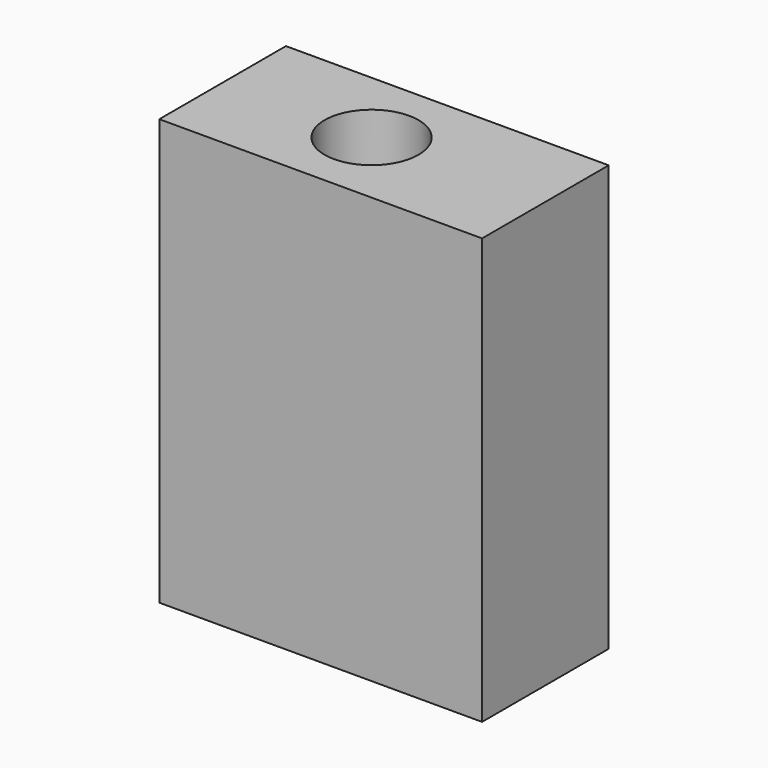
from build123d import *

# Parameters (mm, degrees)
F0_W     = 134.359292686
F0_H     = 65.8905915916
F1_DEPTH = 12.7
F2_W     = 134.359292686
F2_H     = 65.8905915916
F2_R     = 19.5560536298
F3_DEPTH = 151.7965264


# Not quite as in the source:
# - an extrude ends at something that could not be found from the text; its depth is read off the source's solid


with BuildPart() as f1:
    # F0 (on Top) → F1 (new body, symmetric)
    with BuildSketch(Plane.XY):
        with Locations((-0.1394487917, 6.2752943486)):
            Rectangle(F0_W, F0_H)
    extrude(amount=F1_DEPTH, both=True)

    # F2 (on face) → F3 (join, through all)
    with BuildSketch(Plane.XY.offset(12.7)):
        with Locations((-0.1394487917, 6.2752943486)):
            Rectangle(F2_W, F2_H)
        with Locations((-5.4052090272, 6.3866404817)):
            Circle(F2_R, mode=Mode.SUBTRACT)
    extrude(amount=F3_DEPTH)


solid = f1.part
